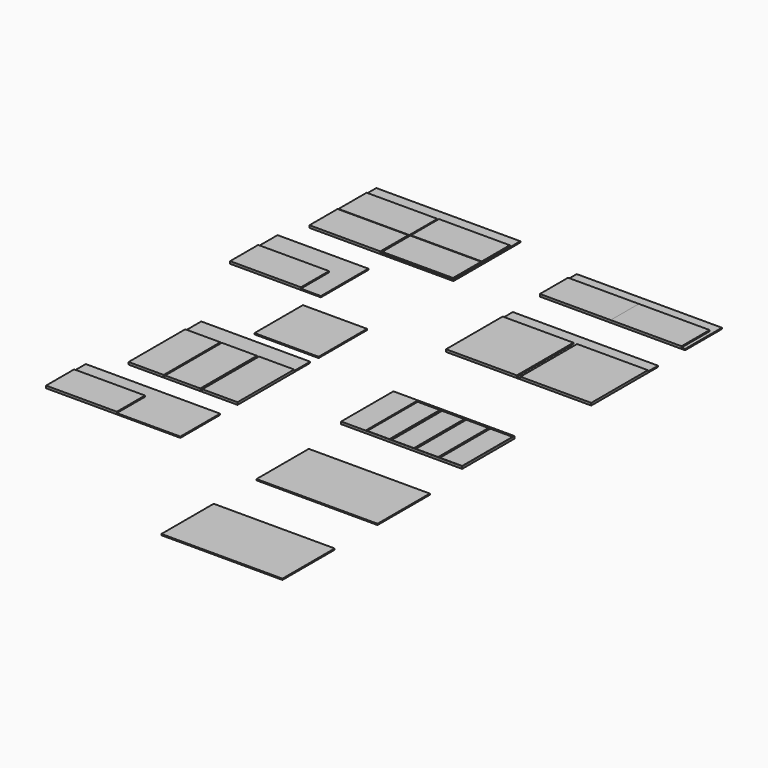
from build123d import *

# Parameters (mm, degrees)
F0_W     = 1190
F0_H     = 690
F2_DEPTH = 10
F0_W_2   = 750
F0_H_2   = 490
F0_W_3   = 530
F0_H_3   = 500
F0_W_4   = 900
F0_H_4   = 750
F0_W_5   = 1110
F0_H_5   = 410
F0_W_6   = 1200
F0_H_6   = 380
F0_W_7   = 1000
F0_H_7   = 540
F3_DEPTH = 10
F1_W     = 290
F1_H     = 585
F1_W_2   = 585
F1_H_2   = 290
F1_W_3   = 1000
F1_H_3   = 540
F1_W_4   = 195
F1_H_4   = 535


# Not quite as in the source:
# - ends of sketch curves that miss each other by under 0.0002 mm in the source are joined


with BuildPart() as f2:
    # F0 (on Top) → F2 (new body)
    with BuildSketch(Plane.XY):
        with Locations((-636.9328212738, 387.6405593753)):
            Rectangle(F0_W, F0_H)
    extrude(amount=-F2_DEPTH)


with BuildPart() as f2b:
    # F0 (on Top) → F2, piece 2 (new body)
    with BuildSketch(Plane.XY):
        with Locations((-943.2546496391, -424.365465641)):
            Rectangle(F0_W_2, F0_H_2)
    extrude(amount=-F2_DEPTH)


with BuildPart() as f2c:
    # F0 (on Top) → F2, piece 3 (new body)
    with BuildSketch(Plane.XY):
        with Locations((-314.3055731058, -1091.1808013916)):
            Rectangle(F0_W_3, F0_H_3)
    extrude(amount=-F2_DEPTH)


with BuildPart() as f2d:
    # F0 (on Top) → F2, piece 4 (new body)
    with BuildSketch(Plane.XY):
        with Locations((-499.3055731058, -1804.1169643402)):
            Rectangle(F0_W_4, F0_H_4)
    extrude(amount=-F2_DEPTH)


with BuildPart() as f2e:
    # F0 (on Top) → F2, piece 5 (new body)
    with BuildSketch(Plane.XY):
        with Locations((-604.3055731058, -2564.4809436798)):
            Rectangle(F0_W_5, F0_H_5)
    extrude(amount=-F2_DEPTH)


with BuildPart() as f2f:
    # F0 (on Top) → F2, piece 6 (new body)
    with BuildSketch(Plane.XY):
        with Locations((1129.5203924179, 411.7811346054)):
            Rectangle(F0_W_6, F0_H_6)
    extrude(amount=-F2_DEPTH)


with BuildPart() as f2g:
    # F0 (on Top) → F2, piece 7 (new body)
    with BuildSketch(Plane.XY):
        with Locations((1139.0423536301, -415.3386044502)):
            Rectangle(F0_W_6, F0_H)
    extrude(amount=-F2_DEPTH)


with BuildPart() as f2h:
    # F0 (on Top) → F2, piece 8 (new body)
    with BuildSketch(Plane.XY):
        with Locations((1141.5956020355, -1702.0453023911)):
            Rectangle(F0_W_7, F0_H_7)
    extrude(amount=-F2_DEPTH)


with BuildPart() as f2i:
    # F0 (on Top) → F2, piece 9 (new body)
    with BuildSketch(Plane.XY):
        with Locations((1205.3639888763, -2656.1429309845)):
            Rectangle(F0_W_7, F0_H_7)
    extrude(amount=-F2_DEPTH)


with BuildPart() as f2j:
    # F0 (on Top) → F2, piece 10 (new body)
    with BuildSketch(Plane.XY):
        with Locations((1205.3639888763, -3638.6525440216)):
            Rectangle(F0_W_7, F0_H_7)
    extrude(amount=-F2_DEPTH)


with BuildPart() as f3:
    # F1 (on Top) → F3 (new body)
    with BuildSketch(Plane.XY):
        Polygon((-642.9328784943, 337.6405584812), (-642.9328784943, 627.6405584812), (-1227.9328784943, 627.6405593753), (-1227.9328784943, 337.6405593753), align=None)
    extrude(amount=F3_DEPTH)


with BuildPart() as f3b:
    # F1 (on Top) → F3, piece 2 (new body)
    with BuildSketch(Plane.XY):
        Polygon((-47.9328799248, 341.6405907273), (-47.9328799248, 631.6405907273), (-632.9328799248, 631.6405907273), (-632.9328799248, 341.6405916214), align=None)
    extrude(amount=F3_DEPTH)


with BuildPart() as f3c:
    # F1 (on Top) → F3, piece 3 (new body)
    with BuildSketch(Plane.XY):
        Polygon((-646.9328784943, 332.6405593753), (-1231.9328784943, 332.6405593753), (-1231.9328212738, 42.6405593753), (-646.9328892231, 42.6405593753), align=None)
    extrude(amount=F3_DEPTH)


with BuildPart() as f3d:
    # F1 (on Top) → F3, piece 4 (new body)
    with BuildSketch(Plane.XY):
        Polygon((-47.9328751564, 335.6405584812), (-632.9328751564, 335.6405584812), (-632.9328751564, 45.6405593753), (-47.9328966141, 45.6405593753), align=None)
    extrude(amount=F3_DEPTH)


with BuildPart() as f3e:
    # F1 (on Top) → F3, piece 5 (new body)
    with BuildSketch(Plane.XY):
        with Locations((-804.3055731058, -1886.6169643402)):
            Rectangle(F1_W, F1_H)
    extrude(amount=F3_DEPTH)


with BuildPart() as f3f:
    # F1 (on Top) → F3, piece 6 (new body)
    with BuildSketch(Plane.XY):
        with Locations((-501.9328999519, -1886.6169643402)):
            Rectangle(F1_W, F1_H)
    extrude(amount=F3_DEPTH)


with BuildPart() as f3g:
    # F1 (on Top) → F3, piece 7 (new body)
    with BuildSketch(Plane.XY):
        Polygon((-49.3055731058, -2179.1169643402), (-49.3055731058, -1594.1169452667), (-339.3055731058, -1594.1169261932), (-339.3055731058, -2179.1169643402), align=None)
    extrude(amount=F3_DEPTH)


with BuildPart() as f3h:
    # F1 (on Top) → F3, piece 8 (new body)
    with BuildSketch(Plane.XY):
        with Locations((-866.8055731058, -2624.4809436798)):
            Rectangle(F1_W_2, F1_H_2)
    extrude(amount=F3_DEPTH)


with BuildPart() as f3i:
    # F1 (on Top) → F3, piece 9 (new body)
    with BuildSketch(Plane.XY):
        Polygon((1114.5203924179, 511.7811346054), (529.5203924179, 511.7811346054), (529.5203924179, 221.7811346054), (1114.5204114914, 221.7811346054), align=None)
    extrude(amount=F3_DEPTH)


with BuildPart() as f3j:
    # F1 (on Top) → F3, piece 10 (new body)
    with BuildSketch(Plane.XY):
        Polygon((1114.5204114914, 221.7811346054), (1699.5204305649, 221.7811346054), (1699.5204305649, 511.7811346054), (1114.5204305649, 511.7811346054), align=None)
    extrude(amount=F3_DEPTH)


with BuildPart() as f3k:
    # F1 (on Top) → F3, piece 11 (new body)
    with BuildSketch(Plane.XY):
        with Locations((831.5423536301, -467.8386044502)):
            Rectangle(F1_W_2, F1_H)
    extrude(amount=F3_DEPTH)


with BuildPart() as f3l:
    # F1 (on Top) → F3, piece 12 (new body)
    with BuildSketch(Plane.XY):
        with Locations((1446.5423536301, -467.8386044502)):
            Rectangle(F1_W_2, F1_H)
    extrude(amount=F3_DEPTH)


with BuildPart() as f3m:
    # F1 (on Top) → F3, piece 13 (new body)
    with BuildSketch(Plane.XY):
        with Locations((1141.5956020355, -1702.0453023911)):
            Rectangle(F1_W_3, F1_H_3)
        with Locations((941.0955572128, -1701.645450592)):
            Rectangle(F1_W_4, F1_H_4, mode=Mode.SUBTRACT)
        with Locations((1143.0952882767, -1701.645450592)):
            Rectangle(F1_W_4, F1_H_4, mode=Mode.SUBTRACT)
        with Locations((1342.9953193665, -1701.6454172134)):
            Rectangle(F1_W_4, F1_H_4, mode=Mode.SUBTRACT)
        with Locations((1541.9953203201, -1701.6454172134)):
            Rectangle(F1_W_4, F1_H_4, mode=Mode.SUBTRACT)
    extrude(amount=F3_DEPTH)


with BuildPart() as f3n:
    # F1 (on Top) → F3, piece 14 (new body)
    with BuildSketch(Plane.XY):
        with Locations((-1025.7546496391, -524.365465641)):
            Rectangle(F1_W_2, F1_H_2)
    extrude(amount=F3_DEPTH)


solid = Compound([f2.part, f2b.part, f2c.part, f2d.part, f2e.part, f2f.part, f2g.part, f2h.part, f2i.part, f2j.part, f3.part, f3b.part, f3c.part, f3d.part, f3e.part, f3f.part, f3g.part, f3h.part, f3i.part, f3j.part, f3k.part, f3l.part, f3m.part, f3n.part])
